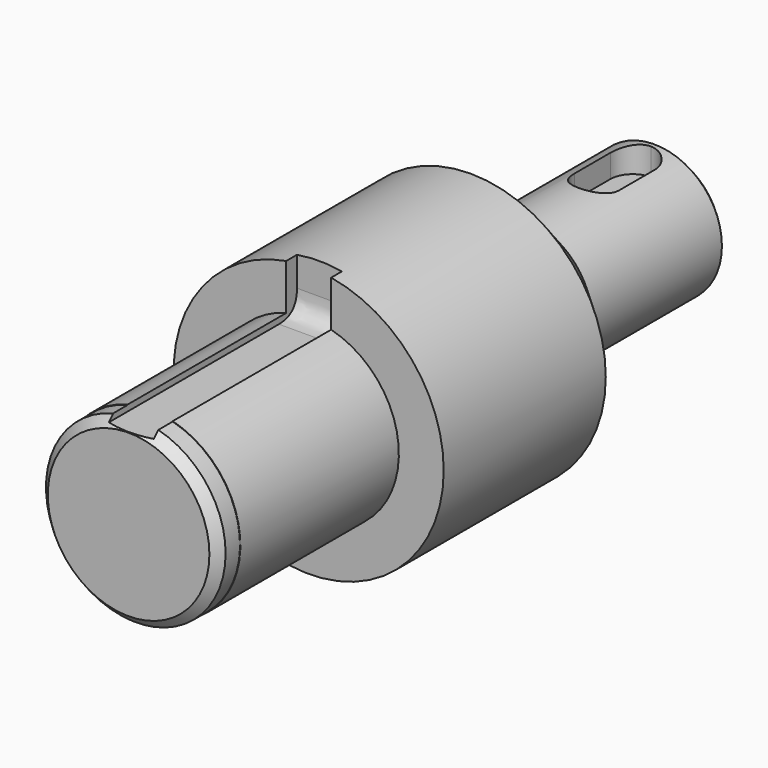
from build123d import *

# Parameters (mm, degrees)
F0_R         = 15
F1_DEPTH     = 74
F2_R         = 15
F2_R_2       = 9.975
F3_DEPTH     = 3
F4_R         = 15
F4_R_2       = 10.0175
F5_DEPTH     = 22
F6_R         = 15
F6_R_2       = 7.5
F7_DEPTH     = 19
F8_SIZE2     = 1
F8_SIZE      = 1
F12_DEPTH    = 26.5
F13_T1_DEPTH = 5
F16_DEPTH    = 3


# Not quite as in the source:
# - a fillet or chamfer that OpenCascade refuses, or shapes differently, is made with other operations: its cross-section is extruded or revolved along the edge and cut away or added


with BuildPart() as f1:
    # F0 (on Front) → F1 (new body)
    with BuildSketch(Plane.XZ):
        Circle(F0_R)
    extrude(amount=F1_DEPTH)

    # F2 (on face) → F3 (cut)
    with BuildSketch(Plane.XZ.offset(74)):
        Circle(F2_R)
        Circle(F2_R_2, mode=Mode.SUBTRACT)
    extrude(amount=-F3_DEPTH, mode=Mode.SUBTRACT)

    # F4 (on face) → F5 (cut)
    with BuildSketch(Plane.XZ.offset(71)):
        Circle(F4_R)
        Circle(F4_R_2, mode=Mode.SUBTRACT)
    extrude(amount=-F5_DEPTH, mode=Mode.SUBTRACT)

    # F6 (on Front) → F7 (cut)
    with BuildSketch(Plane.XZ):
        Circle(F6_R)
        Circle(F6_R_2, mode=Mode.SUBTRACT)
    extrude(amount=F7_DEPTH, mode=Mode.SUBTRACT)

    # F8
    f8_edges = [f1.edges().sort_by_distance(p)[0] for p in [
        (-7.5, 0, 0),
        (-9.975, -74, 0),
    ]]
    chamfer(f8_edges, length=F8_SIZE, length2=F8_SIZE2)

    # F9 (on Right) → F10 (revolve, cut)
    with BuildSketch(Plane.YZ):
        Polygon((-26.5, 15), (-19, 7.5), (-19, 15), align=None)
    revolve(axis=Axis((0, -22.75, 0), (0, 1, 0)), mode=Mode.SUBTRACT)

    # F11 (on face) → F12 (cut)
    with BuildSketch(Plane.XZ.offset(74)):
        with BuildLine():
            Line((-2.5, 14.7901994577), (-2.5, 10.0175))
            Line((-2.5, 10.0175), (-2.5, 9.0175))
            Line((-2.5, 9.0175), (0, 9.0175))
            Line((0, 9.0175), (2.5, 9.0175))
            Line((2.5, 9.0175), (2.5, 10.0175))
            Line((2.5, 10.0175), (2.5, 14.7901994577))
            ThreePointArc((2.5, 14.7901994577), (0, 15), (-2.5, 14.7901994577))
        make_face()
    extrude(amount=-F12_DEPTH, mode=Mode.SUBTRACT)

    # F13: fillet of radius 2.5 on 1 edges, made by hand

    # F13_s2 → F13_t1 (join)
    with BuildSketch(Plane.YZ.offset(-2.5)):
        with BuildLine():
            add(Edge.make_bspline(
                [(-50, 9.0175), (-47.5, 9.0175), (-47.5, 11.5175)],
                knots=[0, 0, 0, 1, 1, 1], degree=2, weights=[1, 1, 1]))
            Line((-47.5, 11.5175), (-47.45, 11.5175))
            Line((-47.45, 11.5175), (-47.45, 8.9675))
            Line((-47.45, 8.9675), (-50, 8.9675))
            Line((-50, 8.9675), (-50, 9.0175))
        make_face()
    extrude(amount=F13_T1_DEPTH)

    # F15 (on offset) → F16 (cut)
    with BuildSketch(Plane.XY.offset(7.5)):
        with BuildLine():
            Line((2.5, -9), (2.5, -4))
            ThreePointArc((2.5, -4), (1.767766953, -2.232233047), (0, -1.5))
            ThreePointArc((0, -1.5), (-1.767766953, -2.232233047), (-2.5, -4))
            Line((-2.5, -4), (-2.5, -9))
            ThreePointArc((-2.5, -9), (-1.767766953, -10.767766953), (0, -11.5))
            ThreePointArc((0, -11.5), (1.767766953, -10.767766953), (2.5, -9))
        make_face()
    extrude(amount=-F16_DEPTH, mode=Mode.SUBTRACT)


solid = f1.part
